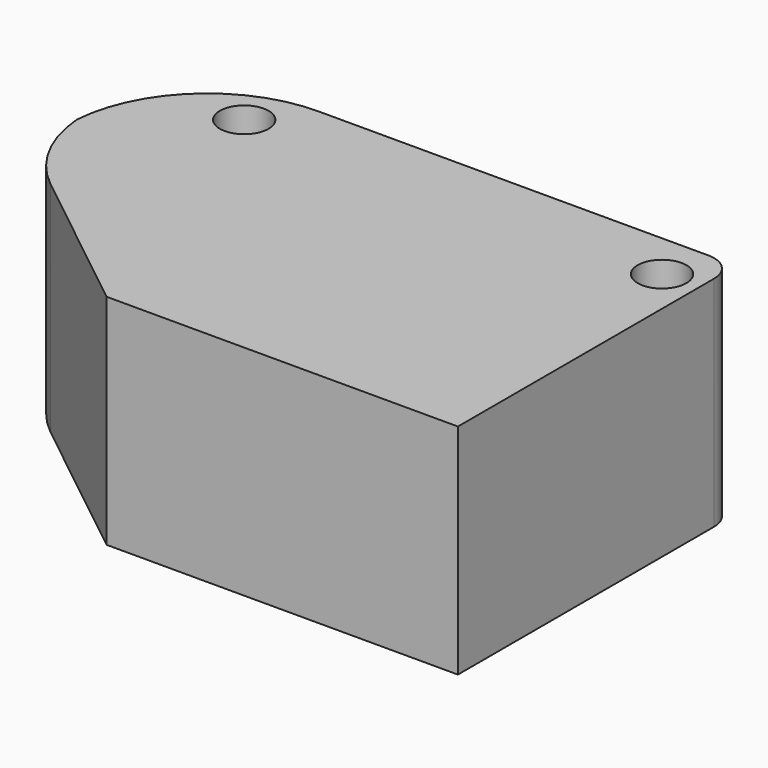
from build123d import *

# Parameters (mm, degrees)
F0_W        = 101.6
F0_H        = 39.83482
F1_DEPTH    = 63.5
F3_DEPTH    = 106.68
F4_T1_DEPTH = 101.2392583659
F4_T3_DEPTH = 166.83482
F5_R        = 5.08
F6_R        = 4.445
F7_DEPTH    = 50.8


# Not quite as in the source:
# - a fillet or chamfer that OpenCascade refuses, or shapes differently, is made with other operations: its cross-section is extruded or revolved along the edge and cut away or added


with BuildPart() as f1:
    # F0 (on Front) → F1 (new body)
    with BuildSketch(Plane.XZ):
        with Locations((-50.8, -19.91741)):
            Rectangle(F0_W, F0_H)
    extrude(amount=F1_DEPTH)

    # F2 (on face) → F3 (cut)
    with BuildSketch(Plane(origin=(0, 0, -39.83482), x_dir=(1, 0, 0), z_dir=(0, 0, -1))):
        Polygon((-101.6, 63.5), (-101.6, 33.7622053921), (-64.0701651573, 63.5), align=None)
    extrude(amount=-F3_DEPTH, mode=Mode.SUBTRACT)

    # F4: fillet of radius 25.4 on 2 edges, made by hand

    # F4_s2 → F4_t1 (cut)
    with BuildSketch(Plane.XY.offset(-70.537039183)):
        with BuildLine():
            ThreePointArc((-91.9745517237, -41.389193495), (-99.0673742894, -32.5376820901), (-101.6, -21.4813177189))
            Line((-101.6, -21.4813177189), (-101.6, -33.7622053921))
            Line((-101.6, -33.7622053921), (-91.9745517237, -41.389193495))
        make_face()
    extrude(amount=F4_T1_DEPTH, mode=Mode.SUBTRACT)

    # F4_s4 → F4_t3 (cut)
    with BuildSketch(Plane.XY.offset(-103.33482)):
        with BuildLine():
            ThreePointArc((-76.2, 0), (-94.1605122421, -7.4394877579), (-101.6, -25.4))
            Line((-101.6, -25.4), (-101.6, 0))
            Line((-101.6, 0), (-76.2, 0))
        make_face()
    extrude(amount=F4_T3_DEPTH, mode=Mode.SUBTRACT)

    # F5
    f5_edges = [f1.edges().sort_by_distance(p)[0] for p in [
        (0, 0, -19.91741),
    ]]
    fillet(f5_edges, radius=F5_R)

    # F6 (on face) → F7 (cut)
    with BuildSketch(Plane(origin=(0, 0, -39.83482), x_dir=(1, 0, 0), z_dir=(0, 0, -1))):
        with Locations((-82.8581005335, 8.6406739429)):
            Circle(F6_R)
        with Locations((-6.6581005335, 8.6406739429)):
            Circle(F6_R)
    extrude(amount=-F7_DEPTH, mode=Mode.SUBTRACT)


solid = f1.part
